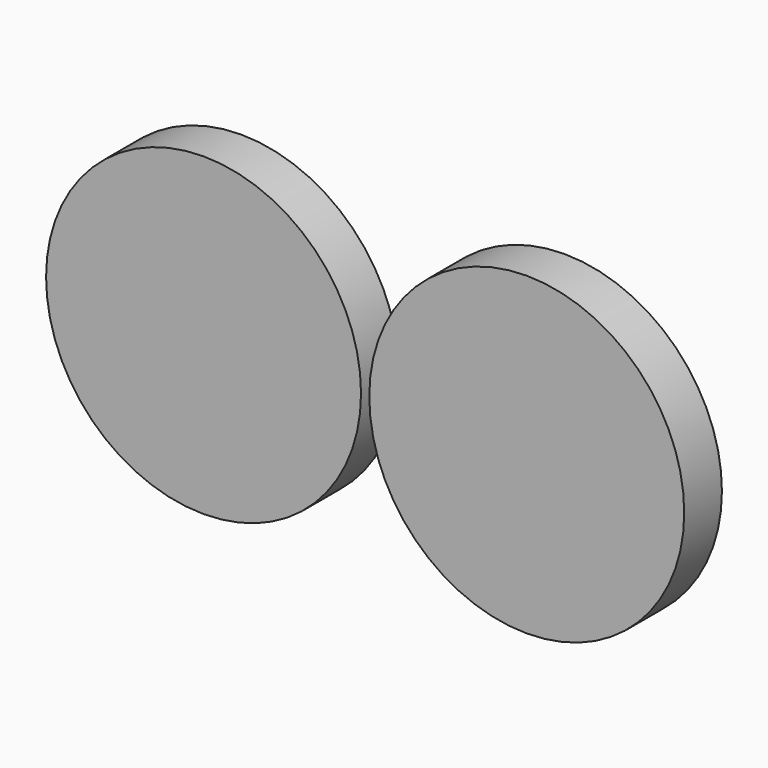
from build123d import *

# Parameters (mm, degrees)
F7_W      = 120
F7_H      = 120
F8_DEPTH  = 15
F9_R      = 50.1388157633
F10_DEPTH = 25


# Not quite as in the source:
# - the program builds the solid bodies; features that only make, move or delete a surface that nothing else refers to are left out


with BuildPart() as f8:
    # F7 (on Front) → F8 (new body)
    with BuildSketch(Plane.XZ):
        with Locations((60.347372832, 60.1354547356)):
            Rectangle(F7_W, F7_H)
        with Locations((-59.652627168, 60.1354547356)):
            Rectangle(F7_W, F7_H)
    extrude(amount=F8_DEPTH)

    # F9 (on face) → F10 (intersect)
    with BuildSketch(Plane.XZ.offset(15)):
        with Locations((51.8001317978, 63.8908669353)):
            Circle(F9_R)
        with Locations((-51.1053861337, 63.8908669353)):
            Circle(F9_R)
    extrude(amount=-F10_DEPTH, mode=Mode.INTERSECT)


solid = f8.part
